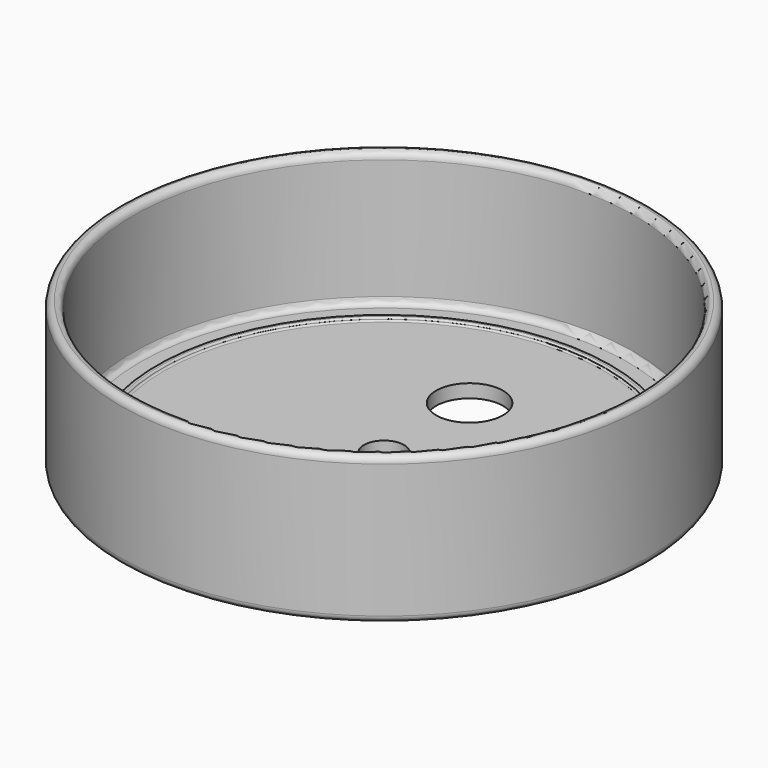
from build123d import *

# Parameters (mm, degrees)
F0_R     = 37.5
F0_R_2   = 5
F0_R_3   = 3
F1_DEPTH = 2
F0_R_4   = 39.5
F2_DEPTH = 22
F3_R     = 34
F3_R_2   = 33.2
F4_DEPTH = 0.5
F5_R     = 0.24999
F6_R     = 0.99999


# Not quite as in the source:
# - a fillet or chamfer is up to 0.001 mm smaller than in the source, because OpenCascade refuses the exact size


with BuildPart() as f1:
    # F0 (on Top) → F1 (new body)
    with BuildSketch(Plane.XY):
        Circle(F0_R)
        with Locations((0, -16)):
            Circle(F0_R_2, mode=Mode.SUBTRACT)
        Circle(F0_R_3, mode=Mode.SUBTRACT)
        with Locations((0, 16)):
            Circle(F0_R_2, mode=Mode.SUBTRACT)
    extrude(amount=F1_DEPTH)

    # F0 (on Top) → F2 (join)
    with BuildSketch(Plane.XY):
        Circle(F0_R_4)
        Circle(F0_R, mode=Mode.SUBTRACT)
    extrude(amount=F2_DEPTH)

    # F3 (on face) → F4 (join)
    with BuildSketch(Plane.XY.offset(2)):
        Circle(F3_R)
        Circle(F3_R_2, mode=Mode.SUBTRACT)
    extrude(amount=F4_DEPTH)

    # F5 (radius 0.25 in the source; OpenCascade refuses exactly that, so slightly less here)
    f5_edges = [f1.edges().sort_by_distance(p)[0] for p in [
        (-34, 0, 2.5),
        (-33.2, 0, 2.5),
        (-33.2, 0, 2),
        (-34, 0, 2),
    ]]
    fillet(f5_edges, radius=F5_R)

    # F6 (radius 1 in the source; OpenCascade refuses exactly that, so slightly less here)
    f6_edges = [f1.edges().sort_by_distance(p)[0] for p in [
        (-37.5, 0, 2),
        (-39.5, 0, 0),
        (-39.5, 0, 22),
        (-37.5, 0, 22),
    ]]
    fillet(f6_edges, radius=F6_R)


solid = f1.part
